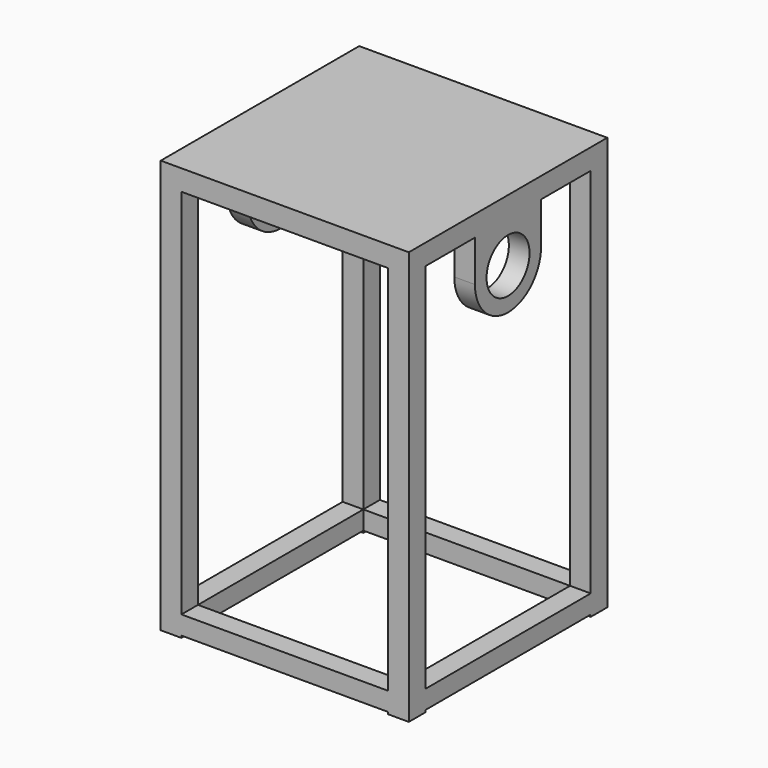
from build123d import *

# Parameters (mm, degrees)
F0_W     = 50
F0_H     = 4.5
F0_R     = 6.5
F1_DEPTH = 60
F4_W     = 50
F4_H     = 50
F5_DEPTH = 4.5
F6_W     = 50
F6_H     = 65
F6_H_2   = 25
F6_H_3   = 0.5
F7_DEPTH = 60


with BuildPart() as f1:
    # F0 (on Right) → F1 (new body)
    with BuildSketch(Plane.YZ):
        Polygon((-55, 95), (-55, 90), (-50, 90), (-35, 90), (-25, 90), (-15, 90), (0, 90), (5, 90), (5, 95), align=None)
        Polygon((-50, 90), (-55, 90), (-55, -5), (-50, -5), (-50, -4.5), (-50, 0), align=None)
        with Locations((-25, -2.25)):
            Rectangle(F0_W, F0_H)
        Polygon((0, 90), (0, 0), (0, -4.5), (0, -5), (5, -5), (5, 90), align=None)
        with BuildLine():
            ThreePointArc((-15, 80), (-17.9289321881, 87.0710678119), (-25, 90))
            ThreePointArc((-25, 90), (-32.0710678119, 87.0710678119), (-35, 80))
            ThreePointArc((-35, 80), (-25, 70), (-15, 80))
        make_face()
        with Locations((-25, 80)):
            Circle(F0_R, mode=Mode.SUBTRACT)
        with BuildLine():
            Line((-25, 90), (-35, 90))
            Line((-35, 90), (-35, 80))
            ThreePointArc((-35, 80), (-32.0710678119, 87.0710678119), (-25, 90))
        make_face()
        with BuildLine():
            Line((-15, 90), (-25, 90))
            ThreePointArc((-25, 90), (-17.9289321881, 87.0710678119), (-15, 80))
            Line((-15, 80), (-15, 90))
        make_face()
    extrude(amount=F1_DEPTH)

    # F4 (on face) → F5 (cut)
    with BuildSketch(Plane(origin=(0, 0, -4.5), x_dir=(1, 0, 0), z_dir=(0, 0, -1))):
        with Locations((30, 25)):
            Rectangle(F4_W, F4_H)
    extrude(amount=-F5_DEPTH, mode=Mode.SUBTRACT)

    # F6 (on offset) → F7 (cut)
    with BuildSketch(Plane.XZ.offset(55)):
        with Locations((30, 57.5)):
            Rectangle(F6_W, F6_H)
        with Locations((30, 12.5)):
            Rectangle(F6_W, F6_H_2)
        with Locations((30, -4.75)):
            Rectangle(F6_W, F6_H_3)
    extrude(amount=-F7_DEPTH, mode=Mode.SUBTRACT)


solid = f1.part
